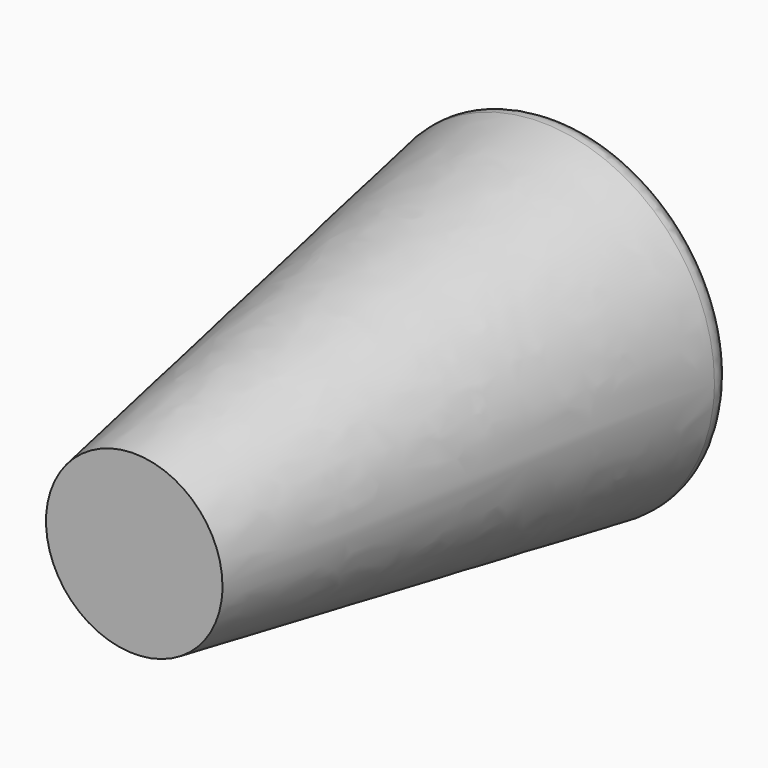
from build123d import *

# Parameters (mm, degrees)
F2_R = 50.8
F3_R = 38.1
F4_R = 25.4
F6_R = 5.08
F7_T = 2.54


# Not quite as in the source:
# - a shell that OpenCascade refuses in one call is made with other operations: the cavity is built on its own and cut out


with BuildPart() as f5:
    # F2 (on Front) → F5 section 0
    with BuildSketch(Plane.XZ):
        Circle(F2_R)
    # F3 (on offset) → F5 section 1
    with BuildSketch(Plane.XZ.offset(76.2)):
        Circle(F3_R)
    # F4 (on offset) → F5 section 2
    with BuildSketch(Plane.XZ.offset(152.4)):
        Circle(F4_R)
    loft()

    # F6
    f6_edges = [f5.edges().sort_by_distance(p)[0] for p in [
        (-50.8, 0, 0),
    ]]
    fillet(f6_edges, radius=F6_R)

    # F7: shell of thickness 2.54, made by hand


with BuildPart() as f7_core1:
    # F7_t2: copy of F5
    add(f5.part)

    # the walls: a layer under each face that stays
    f7_faces = [f7_core1.faces().sort_by_distance(p)[0] for p in [
        (-37.6070710965, -79.1575734206, 0),
        (-48.6794015958, -1.7964155275, 1.2168e-06),
        (2.7e-09, -152.4, -1.5e-09),
    ]]
    thicken(f7_faces, amount=-F7_T, mode=Mode.SUBTRACT)


with BuildPart() as f5_1:
    add(f5.part)

    # what is left inside the walls is the cavity
    f7_cavity = [f7_core1.part.solids().sort_by_distance(p)[0] for p in [
        (-39.263512, -53.614207, 0),
    ]]
    add(f7_cavity, mode=Mode.SUBTRACT)


solid = f5_1.part
